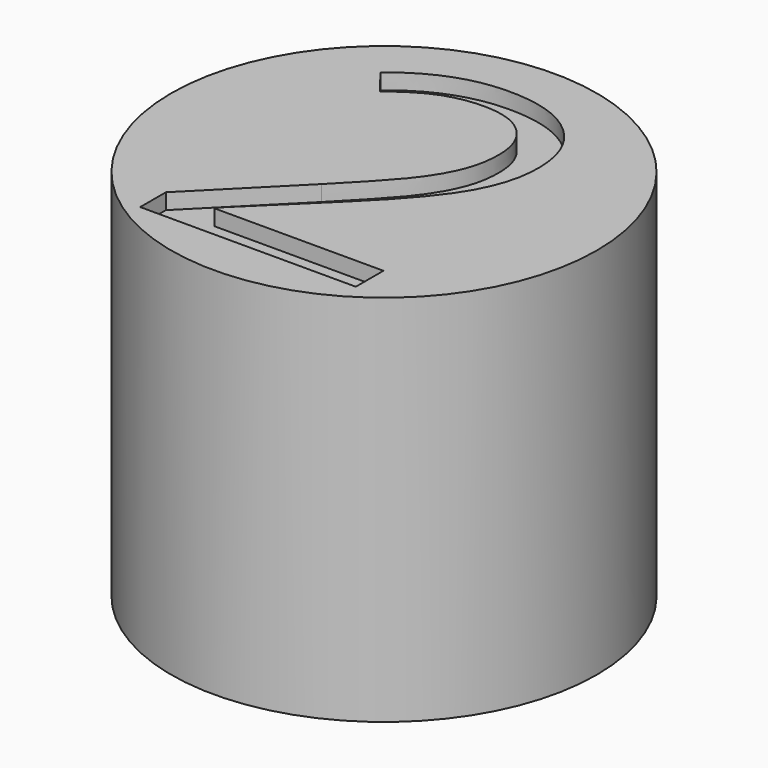
from build123d import *

# Parameters (mm, degrees)
F1_R         = 13.5
F2_DEPTH     = 23.69
F3_TEXT_SIZE = 29.1444731914
F4_DEPTH     = 1


# Not quite as in the source:
# - Text() gives the source's letters only with a copy of the font that has no kerning and outlines rounded to 1/6400 em; it was checked with that copy


with BuildPart() as f2:
    # F1 (on Top) → F2 (new body)
    with BuildSketch(Plane.XY):
        Circle(F1_R)
    extrude(amount=F2_DEPTH)

    # F3 (on face) → F4 (cut)
    with BuildSketch(Plane.XY.offset(23.69)):
        with Locations((-8.4951585529, -10.4920103489)):
            Text('2', F3_TEXT_SIZE, font='Open Sans', text_align=(TextAlign.LEFT, TextAlign.BOTTOM))
    extrude(amount=-F4_DEPTH, mode=Mode.SUBTRACT)


solid = f2.part
